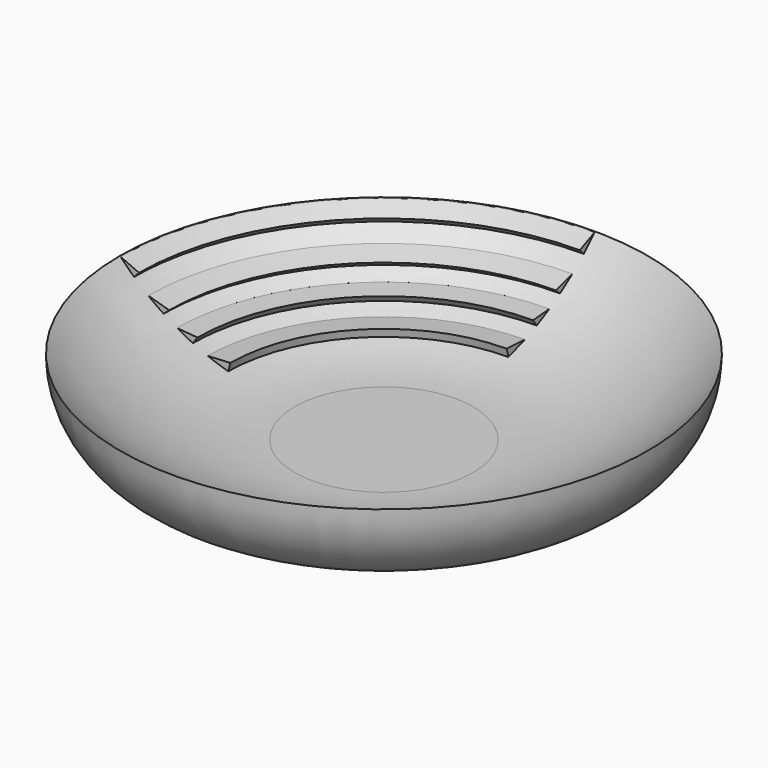
from build123d import *

# Parameters (mm, degrees)
F2_R     = 24.99999
F4_ANGLE = 90


# Not quite as in the source:
# - a fillet or chamfer is up to 0.001 mm smaller than in the source, because OpenCascade refuses the exact size


with BuildPart() as f1:
    # F0 (on Front) → F1 (revolve)
    with BuildSketch(Plane.XZ):
        with BuildLine():
            Line((0, -3.6946386352), (0, 0))
            Line((0, 0), (-25, 0))
            ThreePointArc((-25, 0), (-51.7157183269, 5.5567709647), (-74, 21.3053613648))
            Line((-74, 21.3053613648), (-74, -3.6946386352))
            Line((-74, -3.6946386352), (0, -3.6946386352))
        make_face()
    revolve(axis=Axis((0, 0, -1.8473193176), (0, 0, -1)))

    # F2 (radius 25 in the source; OpenCascade refuses exactly that, so slightly less here)
    f2_edges = [f1.edges().sort_by_distance(p)[0] for p in [
        (74, 0, -3.694639),
    ]]
    fillet(f2_edges, radius=F2_R)

    # F3 (on Front) → F4 (revolve)
    with BuildSketch(Plane.XZ):
        with BuildLine():
            Line((-70.0587433731, 17.3462673245), (-74, 21.2146713292))
            ThreePointArc((-74, 21.2146713292), (-72.0691293591, 19.2399629087), (-70.0587433731, 17.3462673245))
        make_face()
        Polygon((-43.0603352406, 4.9253203614), (-49.4471145262, 4.6049726638), (-43.633293695, 2.6351734955), align=None)
        with BuildLine():
            Line((-43.633293695, 2.6351734955), (-49.4471145262, 4.6049726638))
            ThreePointArc((-49.4471145262, 4.6049726638), (-46.5627090209, 3.5536503103), (-43.633293695, 2.6351734955))
        make_face()
        Polygon((-52.2661279734, 8.1985627052), (-58.0582865363, 8.6943420701), (-53.5528416158, 6.368114131), align=None)
        with BuildLine():
            Line((-53.5528416158, 6.368114131), (-58.0582865363, 8.6943420701))
            ThreePointArc((-58.0582865363, 8.6943420701), (-55.8275138821, 7.4887156535), (-53.5528416158, 6.368114131))
        make_face()
        Polygon((-60.2023862302, 12.3613774776), (-66.1655854553, 14.085889627), (-61.7737689908, 10.9556044658), align=None)
        with BuildLine():
            Line((-61.7737689908, 10.9556044658), (-66.1655854553, 14.085889627))
            ThreePointArc((-66.1655854553, 14.085889627), (-64.001095038, 12.4766675871), (-61.7737689908, 10.9556044658))
        make_face()
        Polygon((-68.6619466735, 18.8474147571), (-74, 21.2146713292), (-70.0587433731, 17.3462673245), align=None)
    revolve(axis=Axis((0, 0, -1.1001997627), (0, 0, -1)), revolution_arc=F4_ANGLE)


solid = f1.part
